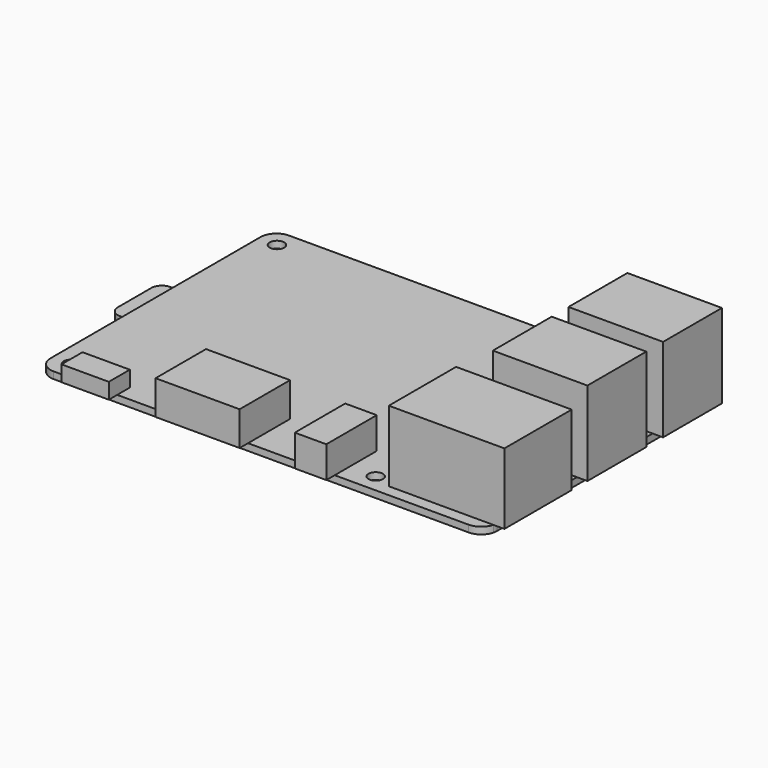
from build123d import *

# Parameters (mm, degrees)
F0_R     = 1.375
F0_W     = 9
F0_H     = 3
F0_W_2   = 16
F0_H_2   = 10
F0_W_3   = 6
F0_H_3   = 14
F1_DEPTH = 1.3
F0_W_4   = 2
F2_DEPTH = 16
F3_DEPTH = 13.5
F0_H_4   = 2
F4_DEPTH = 6
F5_DEPTH = 6.5
F6_DEPTH = 3
F7_W     = 4
F7_H     = 12
F7_W_2   = 12
F8_DEPTH = 3
F9_R     = 2


# Not quite as in the source:
# - a feature names something its author has since deleted; it is built from what else it names


with BuildPart() as f1:
    # F0 (on Top) → F1 (new body)
    with BuildSketch(Plane.XY):
        with BuildLine():
            Line((-28.5, 0), (-3, 0))
            ThreePointArc((-3, 0), (-1.1628826929, 0.6282917549), (-0.0952624903, 2.25))
            Line((-0.0952624903, 2.25), (-20, 2.25))
            Line((-20, 2.25), (-20, 18.25))
            Line((-20, 18.25), (0, 18.25))
            Line((0, 18.25), (0, 22))
            Line((0, 22), (-16, 22))
            Line((-16, 22), (-16, 36))
            Line((-16, 36), (0, 36))
            Line((0, 36), (0, 40))
            Line((0, 40), (-16, 40))
            Line((-16, 40), (-16, 54))
            Line((-16, 54), (-0.1715728753, 54))
            ThreePointArc((-0.1715728753, 54), (-1.2679491924, 55.4494897428), (-3, 56))
            Line((-3, 56), (-82, 56))
            ThreePointArc((-82, 56), (-84.1213203436, 55.1213203436), (-85, 53))
            Line((-85, 53), (-85, 3))
            ThreePointArc((-85, 3), (-84.1213203436, 0.8786796564), (-82, 0))
            Line((-82, 0), (-78.9, 0))
            Line((-78.9, 0), (-78.9, 3))
            Line((-78.9, 3), (-69.9, 3))
            Line((-69.9, 3), (-69.9, 0))
            Line((-69.9, 0), (-61, 0))
            Line((-61, 0), (-61, 10))
            Line((-61, 10), (-45, 10))
            Line((-45, 10), (-45, 0))
            Line((-45, 0), (-34.5, 0))
            Line((-34.5, 0), (-34.5, 10))
            Line((-34.5, 10), (-28.5, 10))
            Line((-28.5, 10), (-28.5, 0))
        make_face()
        with Locations((-81.5, 3.5)):
            Circle(F0_R, mode=Mode.SUBTRACT)
        with Locations((-23.5, 3.5)):
            Circle(F0_R, mode=Mode.SUBTRACT)
        with Locations((-81.5, 52.5)):
            Circle(F0_R, mode=Mode.SUBTRACT)
        with Locations((-23.5, 52.5)):
            Circle(F0_R, mode=Mode.SUBTRACT)
        with Locations((-74.4, 1.5)):
            Rectangle(F0_W, F0_H)
        with Locations((-53, 5)):
            Rectangle(F0_W_2, F0_H_2)
        with Locations((-31.5, 5)):
            Rectangle(F0_W_3, F0_H_2)
        with BuildLine():
            Line((-20, 2.25), (-0.0952624903, 2.25))
            ThreePointArc((-0.0952624903, 2.25), (-0.0239109112, 2.6219871226), (0, 3))
            Line((0, 3), (0, 18.25))
            Line((0, 18.25), (-20, 18.25))
            Line((-20, 18.25), (-20, 2.25))
        make_face()
        with Locations((-8, 29)):
            Rectangle(F0_W_2, F0_H_3)
        with BuildLine():
            Line((-16, 40), (0, 40))
            Line((0, 40), (0, 53))
            ThreePointArc((0, 53), (-0.043204321, 53.5073059362), (-0.1715728753, 54))
            Line((-0.1715728753, 54), (-16, 54))
            Line((-16, 54), (-16, 40))
        make_face()
    extrude(amount=-F1_DEPTH)

    # F0 (on Top) → F2 (join)
    with BuildSketch(Plane.XY):
        with BuildLine():
            Line((-16, 40), (0, 40))
            Line((0, 40), (0, 53))
            ThreePointArc((0, 53), (-0.043204321, 53.5073059362), (-0.1715728753, 54))
            Line((-0.1715728753, 54), (-16, 54))
            Line((-16, 54), (-16, 40))
        make_face()
        with Locations((-8, 29)):
            Rectangle(F0_W_2, F0_H_3)
        with Locations((1, 29)):
            Rectangle(F0_W_4, F0_H_3)
        with BuildLine():
            Line((0, 53), (0, 40))
            Line((0, 40), (2, 40))
            Line((2, 40), (2, 54))
            Line((2, 54), (-0.1715728753, 54))
            ThreePointArc((-0.1715728753, 54), (-0.043204321, 53.5073059362), (0, 53))
        make_face()
    extrude(amount=F2_DEPTH)

    # F0 (on Top) → F3 (join)
    with BuildSketch(Plane.XY):
        with BuildLine():
            Line((-20, 2.25), (-0.0952624903, 2.25))
            ThreePointArc((-0.0952624903, 2.25), (-0.0239109112, 2.6219871226), (0, 3))
            Line((0, 3), (0, 18.25))
            Line((0, 18.25), (-20, 18.25))
            Line((-20, 18.25), (-20, 2.25))
        make_face()
        with BuildLine():
            ThreePointArc((0, 3), (-0.0239109112, 2.6219871226), (-0.0952624903, 2.25))
            Line((-0.0952624903, 2.25), (2, 2.25))
            Line((2, 2.25), (2, 18.25))
            Line((2, 18.25), (0, 18.25))
            Line((0, 18.25), (0, 3))
        make_face()
    extrude(amount=F3_DEPTH)

    # F0 (on Top) → F4 (join)
    with BuildSketch(Plane.XY):
        with Locations((-31.5, -1)):
            Rectangle(F0_W_3, F0_H_4)
        with Locations((-31.5, 5)):
            Rectangle(F0_W_3, F0_H_2)
    extrude(amount=F4_DEPTH)

    # F0 (on Top) → F5 (join)
    with BuildSketch(Plane.XY):
        with Locations((-53, 5)):
            Rectangle(F0_W_2, F0_H_2)
        with Locations((-53, -1)):
            Rectangle(F0_W_2, F0_H_4)
    extrude(amount=F5_DEPTH)

    # F0 (on Top) → F6 (join)
    with BuildSketch(Plane.XY):
        with Locations((-74.4, 1.5)):
            Rectangle(F0_W, F0_H)
        with Locations((-74.4, -1)):
            Rectangle(F0_W, F0_H_4)
    extrude(amount=F6_DEPTH)

    # F7 (on face) → F8 (join)
    with BuildSketch(Plane(origin=(0, 0, -1.3), x_dir=(1, 0, 0), z_dir=(0, 0, -1))):
        with Locations((-87, -28)):
            Rectangle(F7_W, F7_H)
        with Locations((-79, -28)):
            Rectangle(F7_W_2, F7_H)
    extrude(amount=F8_DEPTH)

    # F9
    f9_edges = [f1.edges().sort_by_distance(p)[0] for p in [
        (-89, 22, -2.8),
        (-89, 34, -2.8),
    ]]
    fillet(f9_edges, radius=F9_R)


solid = f1.part
